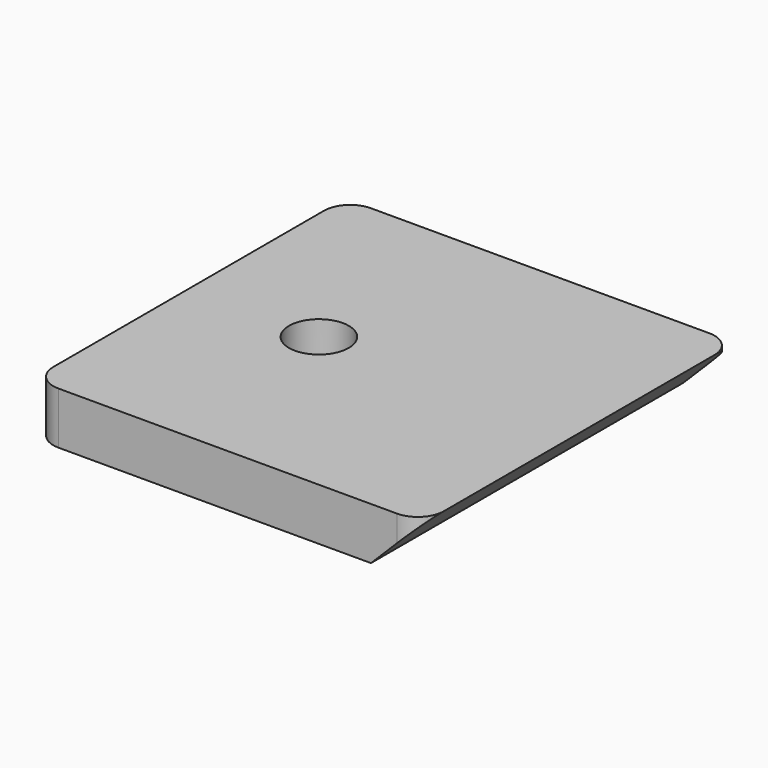
from build123d import *

# Parameters (mm, degrees)
F0_R        = 1.4605
F1_DEPTH    = 2.54
F2_T1_DEPTH = 29.5741495789


# Not quite as in the source:
# - a fillet or chamfer that OpenCascade refuses, or shapes differently, is made with other operations: its cross-section is extruded or revolved along the edge and cut away or added
# - a feature names something its author has since deleted; it is built from what else it names


with BuildPart() as f1:
    # F0 (on Top) → F1 (new body)
    with BuildSketch(Plane.XY):
        with BuildLine():
            Line((-20.32, 2.54), (-3.81, 2.54))
            ThreePointArc((-3.81, 2.54), (-2.9119743879, 2.9119743879), (-2.54, 3.81))
            Line((-2.54, 3.81), (-2.54, 20.32))
            ThreePointArc((-2.54, 20.32), (-2.9119743879, 21.2180256121), (-3.81, 21.59))
            Line((-3.81, 21.59), (-20.32, 21.59))
            ThreePointArc((-20.32, 21.59), (-21.2180256121, 21.2180256121), (-21.59, 20.32))
            Line((-21.59, 20.32), (-21.59, 3.81))
            ThreePointArc((-21.59, 3.81), (-21.2180256121, 2.9119743879), (-20.32, 2.54))
        make_face()
        with Locations((-15.24, 12.065)):
            Circle(F0_R, mode=Mode.SUBTRACT)
    extrude(amount=F1_DEPTH)

    # F2: chamfer of 2.54 on 1 edges, made by hand

    # F2_s2 → F2_t1 (cut)
    with BuildSketch(Plane.XZ.offset(-26.8520747894)):
        Polygon((-2.54, 2.54), (-5.08, 0), (-2.54, 0), align=None)
    extrude(amount=F2_T1_DEPTH, mode=Mode.SUBTRACT)


solid = f1.part
